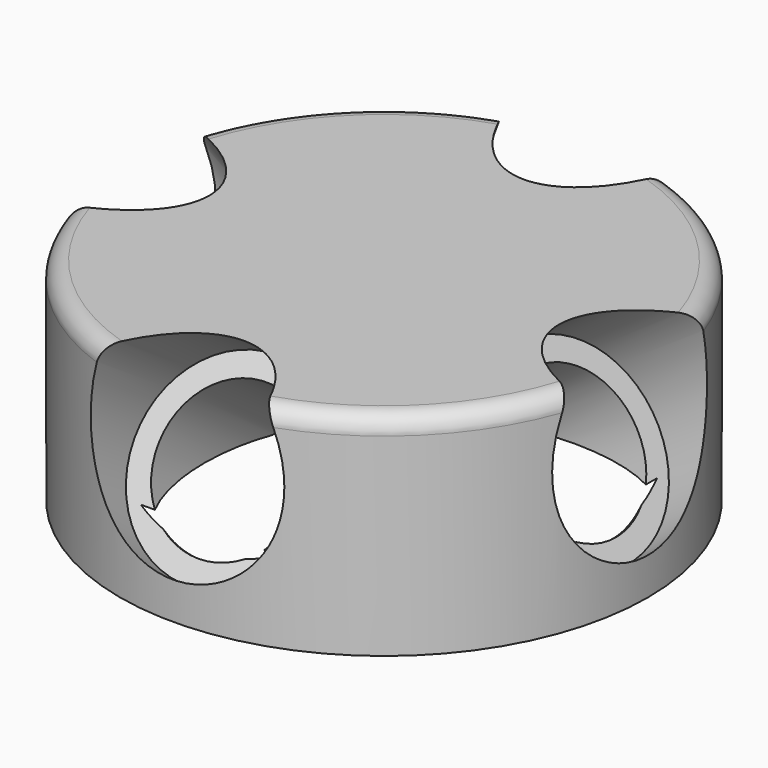
from build123d import *

# Parameters (mm, degrees)
F6_COPIES_COUNT = 4
F7_R            = 1


# Not quite as in the source:
# - a pattern or mirror of a feature is missing from the dataset's text; its kind, count and spacing are read off the source's solid


with BuildPart() as f4:
    # F3 (on Front) → F4 (revolve)
    with BuildSketch(Plane.XZ):
        Polygon((0, 0), (0, 8.46), (-15, 8.46), (-15, -3.54), (-13, -3.54), (-13, 0), align=None)
    revolve(axis=Axis((0, 0, -4.2355582118), (0, 0, -1)))

    # F5 (on Front) → F6 (revolve, cut)
    with BuildSketch(Plane.XZ):
        Polygon((-0.1761714047, -0.0391753335), (-5.0730880905, 3.4278416801), (-8.3376992144, 5.7391863558), (-7.5865121948, 6.800184971), (-14.1157344425, 11.4228743224), (-17.2938333716, 6.9340340271), (-7.5, 0), (-2.5972818806, -3.4588228983), align=None)
    f6 = revolve(axis=Axis((-9.8969166858, 0, 1.6970170136), (-0.816152781, 0, 0.5778361689)), mode=Mode.SUBTRACT)

    # F6_copies: F6 ×4 about axis
    f6_copies_axis = Axis((0, 0, 0), (0, 0, 1))
    for i in range(1, F6_COPIES_COUNT):
        add(f6.rotate(f6_copies_axis, i * 360 / F6_COPIES_COUNT), mode=Mode.SUBTRACT)

    # F7
    f7_edges = [f4.edges().sort_by_distance(p)[0] for p in [
        (-10.606602, 10.606602, 8.46),
        (10.606602, 10.606602, 8.46),
        (10.606602, -10.606602, 8.46),
        (-10.606602, -10.606602, 8.46),
    ]]
    fillet(f7_edges, radius=F7_R)


solid = f4.part
